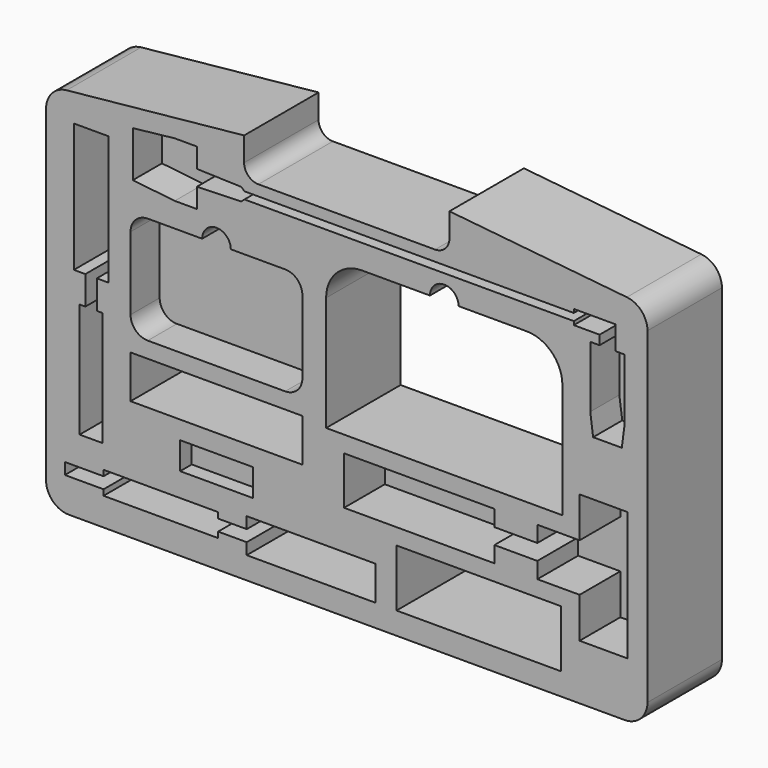
from build123d import *

# Parameters (mm, degrees)
F1_DEPTH  = 65
F11_DEPTH = 65.001
F12_DEPTH = 25.4
F13_DEPTH = 35.56
F9_W      = 120
F9_H      = 30
F8_W      = 115
F8_H      = 40
F14_DEPTH = 65.001
F15_DEPTH = 25.4
F16_DEPTH = 40.64
F10_W     = 50.8
F10_H     = 19.05
F17_DEPTH = 10.16


# Not quite as in the source:
# - a length typed as a fraction of an inch, garbled in the dataset ("3 / 203.2 mm" for 3/8 in), is restored


with BuildPart() as f1:
    # F0 (on Front) → F1 (new body)
    with BuildSketch(Plane.XZ):
        with BuildLine():
            Line((-194, -129.5), (0, -129.5))
            Line((0, -129.5), (194, -129.5))
            ThreePointArc((194, -129.5), (205.313708499, -124.813708499), (210, -113.5))
            Line((210, -113.5), (210, 115.0378975104))
            ThreePointArc((210, 115.0378975104), (205.8697706725, 125.76676251), (195.6114319773, 130.9565434007))
            Line((195.6114319773, 130.9565434007), (71.7, 143.5))
            Line((71.7, 143.5), (71.7, 126.7))
            ThreePointArc((71.7, 126.7), (68.7710678119, 119.6289321881), (61.7, 116.7))
            Line((61.7, 116.7), (0, 116.7))
            Line((0, 116.7), (-61.7, 116.7))
            ThreePointArc((-61.7, 116.7), (-68.7710678119, 119.6289321881), (-71.7, 126.7))
            Line((-71.7, 126.7), (-71.7, 143.5))
            Line((-71.7, 143.5), (-195.6114319773, 130.9565434007))
            ThreePointArc((-195.6114319773, 130.9565434007), (-205.8697706725, 125.76676251), (-210, 115.0378975104))
            Line((-210, 115.0378975104), (-210, -113.5))
            ThreePointArc((-210, -113.5), (-205.313708499, -124.813708499), (-194, -129.5))
        make_face()
    extrude(amount=F1_DEPTH)

    # F10 (on face) → F11 (cut, through all)
    with BuildSketch(Plane.XZ.offset(65)):
        with BuildLine():
            Line((-14.4175440073, -17.7396814525), (55.0347959064, -17.7396814525))
            Line((55.0347959064, -17.7396814525), (150.5824559927, -17.7396814525))
            Line((150.5824559927, -17.7396814525), (150.5824559927, 62.2603185475))
            ThreePointArc((150.5824559927, 62.2603185475), (143.2601255224, 79.9379880772), (125.5824559927, 87.2603185475))
            Line((125.5824559927, 87.2603185475), (78.0824559927, 87.2603185475))
            ThreePointArc((78.0824559927, 87.2603185475), (68.0824559927, 97.2603185475), (58.0824559927, 87.2603185475))
            Line((58.0824559927, 87.2603185475), (10.5824559927, 87.2603185475))
            ThreePointArc((10.5824559927, 87.2603185475), (-7.095213537, 79.9379880772), (-14.4175440073, 62.2603185475))
            Line((-14.4175440073, 62.2603185475), (-14.4175440073, -17.7396814525))
        make_face()
    extrude(amount=-F11_DEPTH, mode=Mode.SUBTRACT)

    # F3 (on face) → F12 (cut)
    with BuildSketch(Plane.XZ.offset(65)):
        with BuildLine():
            ThreePointArc((-151, 7.4711079597), (-147.4852813742, -1.0141734145), (-139, -4.5288920403))
            Line((-139, -4.5288920403), (-101.0147116184, -4.5288920403))
            Line((-101.0147116184, -4.5288920403), (-43, -4.5288920403))
            ThreePointArc((-43, -4.5288920403), (-34.5147186258, -1.0141734145), (-31, 7.4711079597))
            Line((-31, 7.4711079597), (-31, 58.4711079597))
            ThreePointArc((-31, 58.4711079597), (-34.5147186258, 66.956389334), (-43, 70.4711079597))
            Line((-43, 70.4711079597), (-81, 70.4711079597))
            ThreePointArc((-81, 70.4711079597), (-91, 80.4711079597), (-101, 70.4711079597))
            Line((-101, 70.4711079597), (-139, 70.4711079597))
            ThreePointArc((-139, 70.4711079597), (-147.4852813742, 66.956389334), (-151, 58.4711079597))
            Line((-151, 58.4711079597), (-151, 7.4711079597))
        make_face()
    extrude(amount=-F12_DEPTH, mode=Mode.SUBTRACT)

    # F4 (on face) → F13 (cut)
    with BuildSketch(Plane.XZ.offset(65)):
        Polygon((162.6070588827, -90.9896814525), (196.1070588827, -90.9896814525), (196.1070588827, -45.9896814525), (196.1070588827, -0.9896814525), (162.6070588827, -0.9896814525), (162.6070588827, -29.2396814525), (133.1070588827, -29.2396814525), (133.1070588827, -40.4896814525), (103.1070588827, -40.4896814525), (103.1070588827, -29.2396814525), (-1.8929411173, -29.2396814525), (-1.8929411173, -45.9896814525), (-1.8929411173, -62.7396814525), (103.1070588827, -62.7396814525), (103.1070588827, -51.4896814525), (133.1070588827, -51.4896814525), (133.1070588827, -62.7396814525), (162.6070588827, -62.7396814525), align=None)
    extrude(amount=-F13_DEPTH, mode=Mode.SUBTRACT)

    # F9 (on face) + F8 (on face) → F14 (cut, through all)
    with BuildSketch(Plane.XZ.offset(65)):
        with Locations((-91, -30.7038457692)):
            Rectangle(F9_W, F9_H)
    with BuildSketch(Plane.XZ.offset(65)):
        with Locations((92.2330532188, -93.9844995737)):
            Rectangle(F8_W, F8_H)
    extrude(amount=-F14_DEPTH, mode=Mode.SUBTRACT)

    # F7 (on face) → F15 (cut)
    with BuildSketch(Plane.XZ.offset(65)):
        Polygon((-149.4115442038, 122.7246001363), (-149.4115442038, 106.7246001363), (-149.4115442038, 90.7246001363), (-120.1630565758, 87.4952884788), (-104.6630565758, 87.4952884788), (-104.6630565758, 101.2452884788), (-73.6785290068, 102.2246001363), (-71.4424610293, 104.2246001363), (158.5575389707, 104.2246001363), (158.5575389707, 101.7246001363), (176.5575389707, 101.7246001363), (176.5575389707, 95.2246001363), (170.0575389707, 95.2246001363), (170.0575389707, 52.2246001363), (172.0575389707, 37.2246001363), (182.0575389707, 37.2246001363), (192.0575389707, 37.2246001363), (194.0575389707, 52.2246001363), (194.0575389707, 95.2246001363), (187.5575389707, 95.2246001363), (187.5575389707, 111.7246001363), (158.5575389707, 111.7246001363), (158.5575389707, 109.2246001363), (-71.4424610293, 109.2246001363), (-73.6785290068, 111.2246001363), (-104.6630565758, 112.2039117938), (-104.6630565758, 125.9539117938), (-120.1630565758, 125.9539117938), align=None)
    extrude(amount=-F15_DEPTH, mode=Mode.SUBTRACT)

    # F7 (on face) + F5 (on face) → F16 (cut)
    with BuildSketch(Plane.XZ.offset(65)):
        Polygon((-89.8567122221, -93.9844995737), (-169.8567122221, -93.9844995737), (-169.8567122221, -97.9844995737), (-196.8567122221, -97.9844995737), (-196.8567122221, -101.9844995737), (-196.8567122221, -105.9844995737), (-169.8567122221, -105.9844995737), (-169.8567122221, -109.9844995737), (-89.8567122221, -109.9844995737), (-89.8567122221, -105.9844995737), (-69.8567122221, -105.9844995737), (-69.8567122221, -113.9844995737), (20.1432877779, -113.9844995737), (20.1432877779, -101.9844995737), (20.1432877779, -89.9844995737), (-69.8567122221, -89.9844995737), (-69.8567122221, -97.9844995737), (-89.8567122221, -97.9844995737), align=None)
    with BuildSketch(Plane.XZ.offset(65)):
        Polygon((-186.5798817873, 2.1856421232), (-186.5798817873, -77.8143578768), (-178.5798817873, -77.8143578768), (-170.5798817873, -77.8143578768), (-170.5798817873, 2.1856421232), (-174.5798817873, 2.1856421232), (-174.5798817873, 22.1856421232), (-166.5798817873, 22.1856421232), (-166.5798817873, 112.1856421232), (-178.5798817873, 112.1856421232), (-190.5798817873, 112.1856421232), (-190.5798817873, 22.1856421232), (-182.5798817873, 22.1856421232), (-182.5798817873, 2.1856421232), align=None)
    extrude(amount=-F16_DEPTH, mode=Mode.SUBTRACT)

    # F10 (on face) → F17 (cut)
    with BuildSketch(Plane.XZ.offset(65)):
        with Locations((-91, -67.9338675678)):
            Rectangle(F10_W, F10_H)
    extrude(amount=-F17_DEPTH, mode=Mode.SUBTRACT)


solid = f1.part
